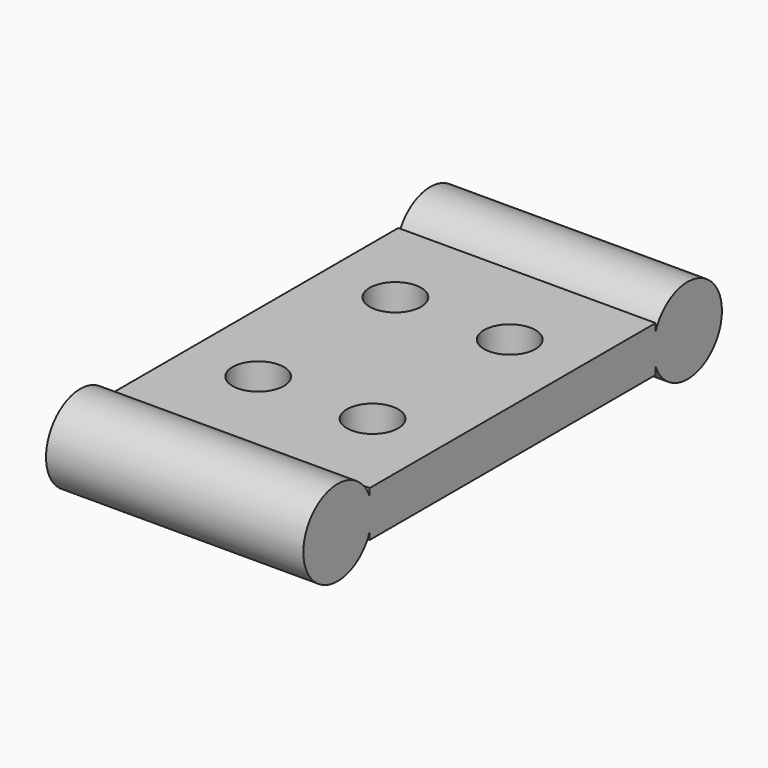
from build123d import *

# Parameters (mm, degrees)
F0_W     = 45
F0_H     = 62.5
F1_DEPTH = 8
F3_D     = 9
F3_DEPTH = 15
F3_TIP   = 2.7038727856
F5_DEPTH = 45


with BuildPart() as f1:
    # F0 (on Top) → F1 (new body)
    with BuildSketch(Plane.XY):
        with Locations((22.5, -31.25)):
            Rectangle(F0_W, F0_H)
    extrude(amount=F1_DEPTH)

    # F3
    with Locations(Plane.XY.offset(8)):
        with Locations((12.5, -16.25), (32.5, -16.25), (32.5, -46.25), (12.5, -46.25)):
            Hole(F3_D / 2, depth=F3_DEPTH)
            with Locations((0, 0, -(F3_DEPTH + F3_TIP / 2))):  # 118° drill point
                Cone(0, F3_D / 2, F3_TIP, mode=Mode.SUBTRACT)

    # F4 (on face) → F5 (join)
    with BuildSketch(Plane.YZ.offset(45)):
        with BuildLine():
            ThreePointArc((-62.5, 1.3074175964), (-62.1260593981, 2.6306936062), (-62, 4))
            ThreePointArc((-62, 4), (-62.1260593981, 5.3693063938), (-62.5, 6.6925824036))
            Line((-62.5, 6.6925824036), (-62.5, 1.3074175964))
        make_face()
        with BuildLine():
            Line((-62.5, 1.3074175964), (-62.5, 6.6925824036))
            ThreePointArc((-62.5, 6.6925824036), (-77, 4), (-62.5, 1.3074175964))
        make_face()
        with BuildLine():
            ThreePointArc((14.5, 4), (8.3693063938, 11.3739406019), (0, 6.6925824036))
            Line((0, 6.6925824036), (0, 1.3074175964))
            ThreePointArc((0, 1.3074175964), (8.3693063938, -3.3739406019), (14.5, 4))
        make_face()
    extrude(amount=-F5_DEPTH)


solid = f1.part
